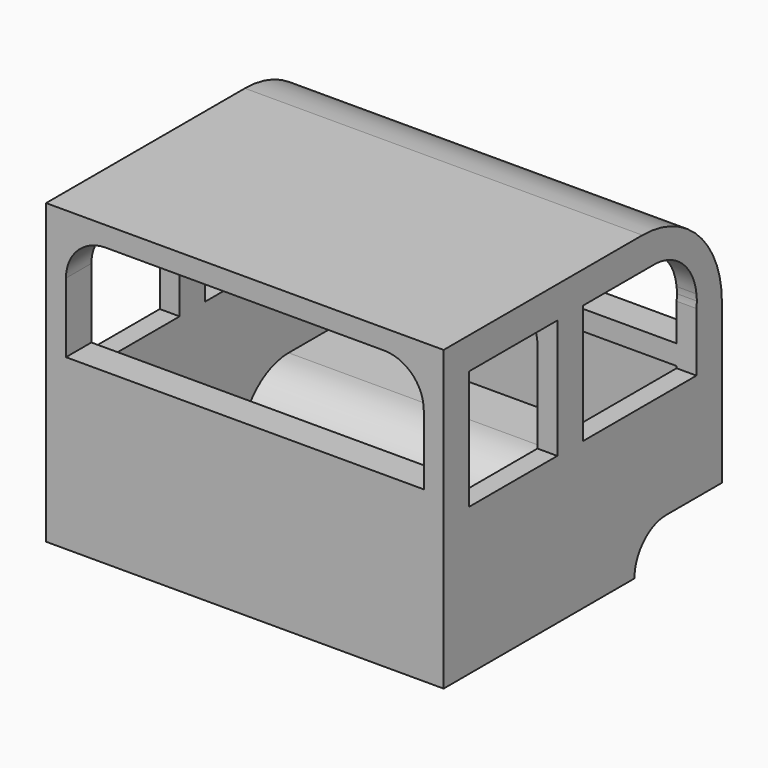
from build123d import *

# Parameters (mm, degrees)
F0_W         = 50.8
F0_H         = 44.45
F1_DEPTH     = 38.1
F2_W         = 13.97
F2_H         = 5.08
F3_DEPTH     = 50.8
F4_R         = 12.7
F5_W         = 45.72
F5_H         = 13.97
F6_DEPTH     = 50.8
F7_R         = 5.08
F8_W         = 14.097
F8_H         = 15.24
F9_DEPTH     = 50.8
F10_R        = 5.07999
F11_T        = 2.54
F11_T3_DEPTH = 9.0721543583
F11_T5_DEPTH = 9.0721543583
F11_T7_DEPTH = 9.144
F11_T9_DEPTH = 9.144


# Not quite as in the source:
# - a fillet or chamfer is up to 0.001 mm smaller than in the source, because OpenCascade refuses the exact size
# - a shell that OpenCascade refuses in one call is made with other operations: the cavity is built on its own and cut out


with BuildPart() as f1:
    # F0 (on Top) → F1 (new body)
    with BuildSketch(Plane.XY):
        Rectangle(F0_W, F0_H)
    extrude(amount=F1_DEPTH)

    # F2 (on face) → F3 (cut)
    with BuildSketch(Plane.YZ.offset(25.4)):
        with Locations((15.24, 2.54)):
            Rectangle(F2_W, F2_H)
    extrude(amount=-F3_DEPTH, mode=Mode.SUBTRACT)

    # F4
    f4_edges = [f1.edges().sort_by_distance(p)[0] for p in [
        (0, 22.225, 38.1),
    ]]
    fillet(f4_edges, radius=F4_R)

    # F5 (on face) → F6 (cut)
    with BuildSketch(Plane(origin=(0, 22.225, 0), x_dir=(-1, 0, 0), z_dir=(0, 1, 0))):
        with Locations((0, 28.575)):
            Rectangle(F5_W, F5_H)
    extrude(amount=-F6_DEPTH, mode=Mode.SUBTRACT)

    # F7
    f7_edges = [f1.edges().sort_by_distance(p)[0] for p in [
        (22.86, -2.54, 35.56),
        (-22.86, -2.54, 35.56),
    ]]
    fillet(f7_edges, radius=F7_R)

    # F8 (on face) → F9 (cut)
    with BuildSketch(Plane.YZ.offset(25.4)):
        with BuildLine():
            ThreePointArc((18.161, 26.3400295448), (18.1977232283, 26.7491865029), (18.2099788483, 27.1598053184))
            ThreePointArc((18.2099788483, 27.1598053184), (18.1977232283, 27.5704241338), (18.161, 27.9795810919))
            Line((18.161, 27.9795810919), (18.161, 26.3400295448))
        make_face()
        with BuildLine():
            Line((18.161, 26.3400295448), (18.161, 27.9795810919))
            ThreePointArc((18.161, 27.9795810919), (15.7632997742, 32.4232792644), (10.978474631, 34.036))
            ThreePointArc((10.978474631, 34.036), (6.2916716696, 22.46222933), (18.161, 26.3400295448))
        make_face()
        with BuildLine():
            Line((18.161, 18.796), (18.161, 26.3400295448))
            ThreePointArc((18.161, 26.3400295448), (6.2916716696, 22.46222933), (10.978474631, 34.036))
            Line((10.978474631, 34.036), (0, 34.036))
            Line((0, 34.036), (0, 18.796))
            Line((0, 18.796), (18.161, 18.796))
        make_face()
        with Locations((-11.1125, 26.416)):
            Rectangle(F8_W, F8_H)
    extrude(amount=-F9_DEPTH, mode=Mode.SUBTRACT)

    # F10 (radius 5.08 in the source; OpenCascade refuses exactly that, so slightly less here)
    f10_edges = [f1.edges().sort_by_distance(p)[0] for p in [
        (0, 8.255, 5.08),
    ]]
    fillet(f10_edges, radius=F10_R)

    # F11: shell of thickness 2.54, made by hand


with BuildPart() as f11_core1:
    # F11_t2: copy of F1
    add(f1.part)

    # the walls: a layer under each face that stays
    f11_faces = [f11_core1.faces().sort_by_distance(p)[0] for p in [
        (-25.4, 14.8166666667, 6.35),
        (0, 17.779995, 5.08),
        (0, 9.7428946226, 3.5921053774),
        (0, 22.225, 15.24),
        (0, 8.255, 5e-06),
        (16.9333333333, 12.8120018728, 37.6672579939),
        (0, -6.985, 0),
        (0, -6.35, 38.1),
        (0, -22.225, 19.05),
        (-23.4039228208, 5.4892373155, 34.036),
        (-23.3996024836, 16.3584390419, 31.8573813067),
        (-23.4039228208, -11.1125, 34.036),
        (-16.9333333333, -18.161, 21.336),
        (25.4, -14.8166666667, 6.35),
        (-22.86, 19.7907563947, 26.035),
        (0, 20.193, 21.59),
        (22.86, 19.7907563947, 26.035),
        (-21.3721024484, -0.5301288674, 34.0721024484),
        (0, -2.54, 35.56),
        (21.3721024484, -0.5301288674, 34.0721024484),
        (22.86, -20.193, 26.035),
        (0, -20.193, 21.59),
        (-22.86, -20.193, 26.035),
        (-22.86, -2.032, 26.035),
        (22.86, -2.032, 26.035),
        (23.4039228208, 5.4892373155, 34.036),
        (23.3996024836, 16.3584390419, 31.8573813067),
        (23.4039228208, -11.1125, 34.036),
    ]]
    thicken(f11_faces, amount=-F11_T, mode=Mode.SUBTRACT)

    # F11_s4 → F11_t3 (cut)
    with BuildSketch(Plane.YZ.offset(-27.94)):
        Polygon((-18.1356, 34.0106), (-18.161, 36.576), (-20.701, 36.576), (-20.701, 34.036), align=None)
    extrude(amount=F11_T3_DEPTH, mode=Mode.SUBTRACT)

    # F11_s6 → F11_t5 (cut)
    with BuildSketch(Plane.YZ.offset(18.8678456417)):
        Polygon((-18.1356, 34.0106), (-20.701, 34.036), (-20.701, 36.576), (-18.161, 36.576), align=None)
    extrude(amount=F11_T5_DEPTH, mode=Mode.SUBTRACT)

    # F11_s8 → F11_t7 (cut)
    with BuildSketch(Plane.XZ.offset(-24.765)):
        Polygon((-22.8346, 21.6154), (-25.4, 21.59), (-25.4, 19.05), (-22.86, 19.05), align=None)
        Polygon((22.8346, 21.6154), (22.86, 19.05), (25.4, 19.05), (25.4, 21.59), align=None)
    extrude(amount=F11_T7_DEPTH, mode=Mode.SUBTRACT)

    # F11_s10 → F11_t9 (cut)
    with BuildSketch(Plane.XZ.offset(15.621)):
        Polygon((22.8346, 21.6154), (25.4, 21.59), (25.4, 19.05), (22.86, 19.05), align=None)
        Polygon((-22.8346, 21.6154), (-22.86, 19.05), (-25.4, 19.05), (-25.4, 21.59), align=None)
    extrude(amount=F11_T9_DEPTH, mode=Mode.SUBTRACT)


with BuildPart() as f1_1:
    add(f1.part)

    # what is left inside the walls is the cavity
    f11_cavity = [f11_core1.part.solids().sort_by_distance(p)[0] for p in [
        (0, -11.073069, 2.5654),
    ]]
    add(f11_cavity, mode=Mode.SUBTRACT)


solid = f1_1.part
